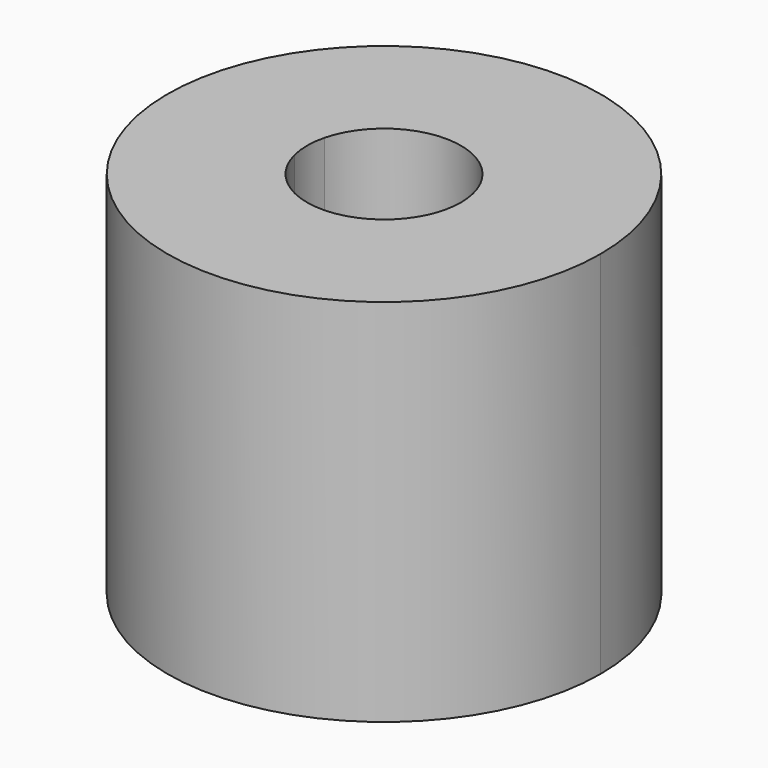
from build123d import *

# Parameters (mm, degrees)
F2_DEPTH = 25.4


with BuildPart() as f2:
    # F1 (on face) → F2 (new body)
    with BuildSketch(Plane.XY):
        with BuildLine():
            ThreePointArc((-4.8808341445, 14.0525419265), (-5.004069886, 14.0091313477), (-5.1269195974, 13.9646400592))
            Line((-5.1269195974, 13.9646400592), (-5.1269195974, 1.288408295))
            ThreePointArc((-5.1269195974, 1.288408295), (-1.4388144753, 5.0867586338), (3.6924446467, 3.783008462))
            Line((3.6924446467, 3.783008462), (3.6924446467, 14.4104937137))
            ThreePointArc((3.6924446467, 14.4104937137), (3.6125240495, 14.4307361744), (3.5324924947, 14.450535399))
            Line((3.5324924947, 14.450535399), (3.0549003277, 14.0525419265))
            Line((3.0549003277, 14.0525419265), (-4.8808341445, 14.0525419265))
        make_face()
        with BuildLine():
            Line((-5.1269195974, 1.288408295), (-5.1269195974, 13.9646400592))
            ThreePointArc((-5.1269195974, 13.9646400592), (-8.5155220323, -12.1976375196), (14.8760369905, 0))
            ThreePointArc((14.8760369905, 0), (11.752136395, 9.1205135105), (3.6924446467, 14.4104937137))
            Line((3.6924446467, 14.4104937137), (3.6924446467, 3.783008462))
            ThreePointArc((3.6924446467, 3.783008462), (4.8715904415, 2.0525367386), (5.2863314778, 0))
            ThreePointArc((5.2863314778, 0), (4.8715904415, -2.0525367386), (3.6924446467, -3.783008462))
            Line((3.6924446467, -3.783008462), (3.6924446467, -11.555492878))
            Line((3.6924446467, -11.555492878), (-4.7550187446, -10.9179485589))
            Line((-4.7550187446, -10.9179485589), (-5.1269195974, -10.9179485589))
            Line((-5.1269195974, -10.9179485589), (-5.1269195974, -1.288408295))
            ThreePointArc((-5.1269195974, -1.288408295), (-5.2863314778, 0), (-5.1269195974, 1.288408295))
        make_face()
        with BuildLine():
            ThreePointArc((3.5324924947, 14.450535399), (-0.7029267403, 14.8594202626), (-4.8808341445, 14.0525419265))
            Line((-4.8808341445, 14.0525419265), (3.0549003277, 14.0525419265))
            Line((3.0549003277, 14.0525419265), (3.5324924947, 14.450535399))
        make_face()
        with BuildLine():
            ThreePointArc((3.6924446467, -3.783008462), (-1.4388144753, -5.0867586338), (-5.1269195974, -1.288408295))
            Line((-5.1269195974, -1.288408295), (-5.1269195974, -10.9179485589))
            Line((-5.1269195974, -10.9179485589), (-4.7550187446, -10.9179485589))
            Line((-4.7550187446, -10.9179485589), (3.6924446467, -11.555492878))
            Line((3.6924446467, -11.555492878), (3.6924446467, -3.783008462))
        make_face()
    extrude(amount=F2_DEPTH)


solid = f2.part
